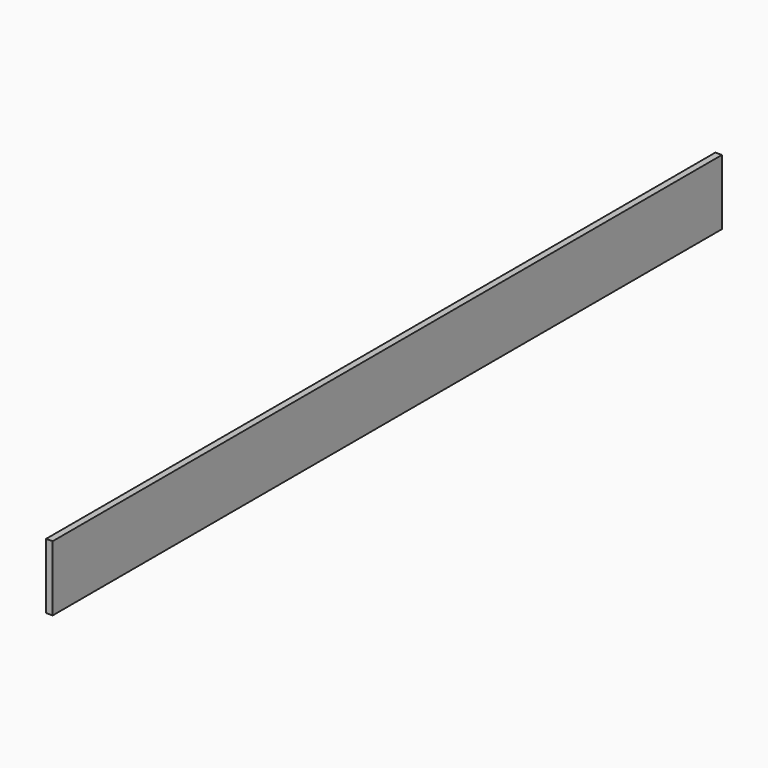
from build123d import *

# Parameters (mm, degrees)
F0_W     = 10
F0_H     = 100
F1_DEPTH = 1280


# Not quite as in the source:
# - a feature names something its author has since deleted; it is built from what else it names


with BuildPart() as f1:
    # F0 (on Front) → F1 (new body)
    with BuildSketch(Plane.XZ):
        with Locations((5, 50)):
            Rectangle(F0_W, F0_H)
    extrude(amount=F1_DEPTH)


solid = f1.part
